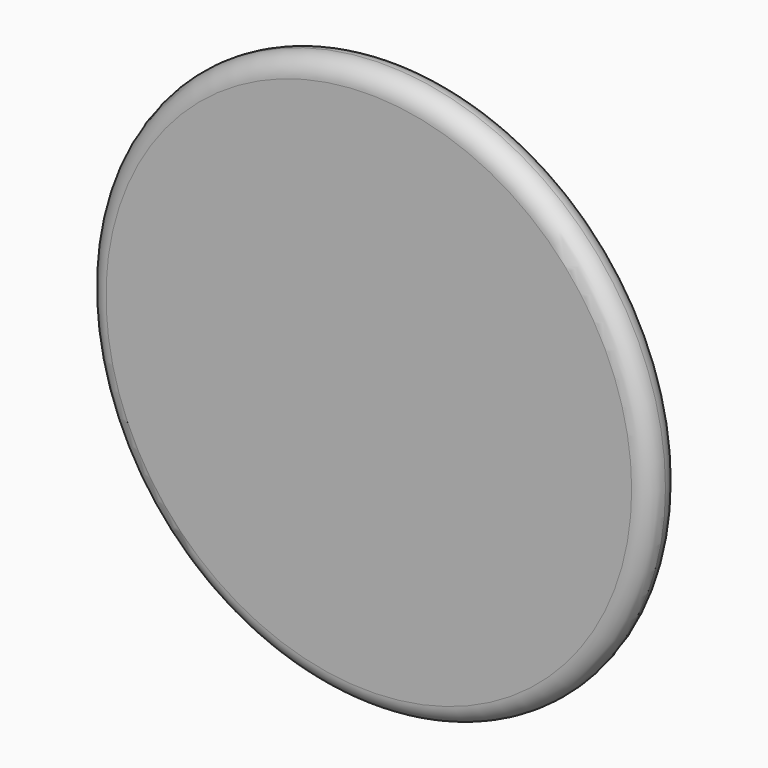
from build123d import *

# Parameters (mm, degrees)
F0_R     = 15
F1_DEPTH = 2
F2_R     = 0.99999


# Not quite as in the source:
# - a fillet or chamfer is up to 0.001 mm smaller than in the source, because OpenCascade refuses the exact size


with BuildPart() as f1:
    # F0 (on Front) → F1 (new body)
    with BuildSketch(Plane.XZ):
        Circle(F0_R)
    extrude(amount=F1_DEPTH)

    # F2 (radius 1 in the source; OpenCascade refuses exactly that, so slightly less here)
    f2_edges = [f1.edges().sort_by_distance(p)[0] for p in [
        (-15, -2, 0),
        (-15, 0, 0),
    ]]
    fillet(f2_edges, radius=F2_R)


solid = f1.part
